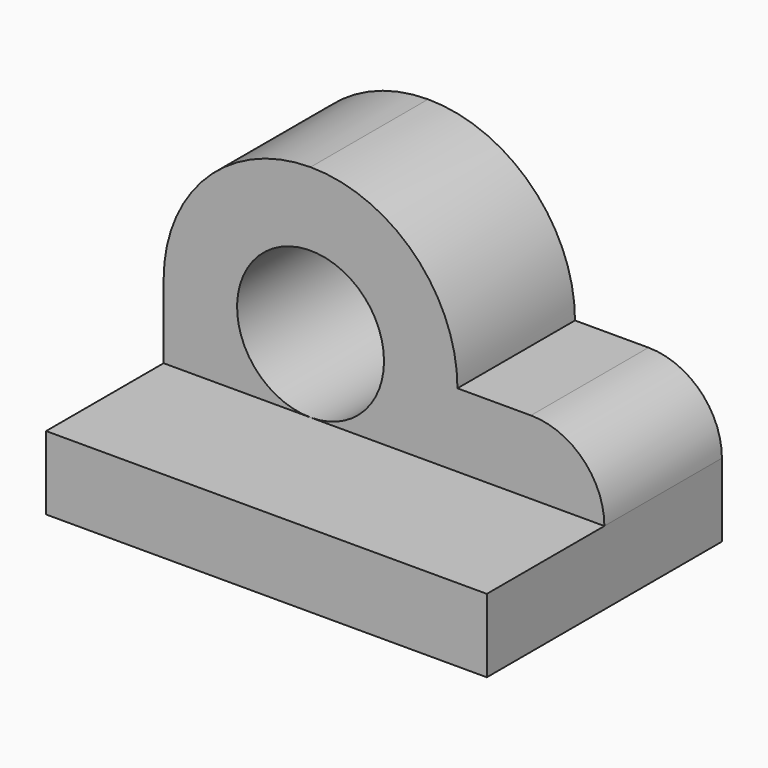
from build123d import *

# Parameters (mm, degrees)
F0_W     = 60
F0_H     = 10
F1_DEPTH = 40
F2_W     = 60
F2_H     = 20
F3_DEPTH = 10
F4_W     = 40
F4_H     = 20
F5_DEPTH = 20
F6_R     = 19.99999
F7_R     = 10
F8_R     = 10
F9_DEPTH = 25


# Not quite as in the source:
# - a fillet or chamfer is up to 0.001 mm smaller than in the source, because OpenCascade refuses the exact size


with BuildPart() as f1:
    # F0 (on Front) → F1 (new body)
    with BuildSketch(Plane.XZ):
        with Locations((30, 5)):
            Rectangle(F0_W, F0_H)
    extrude(amount=F1_DEPTH)

    # F2 (on face) → F3 (join)
    with BuildSketch(Plane.XY.offset(10)):
        with Locations((30, -10)):
            Rectangle(F2_W, F2_H)
    extrude(amount=F3_DEPTH)

    # F4 (on face) → F5 (join)
    with BuildSketch(Plane.XY.offset(20)):
        with Locations((20, -10)):
            Rectangle(F4_W, F4_H)
    extrude(amount=F5_DEPTH)

    # F6 (radius 20 in the source; OpenCascade refuses exactly that, so slightly less here)
    f6_edges = [f1.edges().sort_by_distance(p)[0] for p in [
        (0, -10, 40),
        (40, -10, 40),
    ]]
    fillet(f6_edges, radius=F6_R)

    # F7
    f7_edges = [f1.edges().sort_by_distance(p)[0] for p in [
        (60, -10, 20),
    ]]
    fillet(f7_edges, radius=F7_R)

    # F8 (on face) → F9 (cut)
    with BuildSketch(Plane.XZ.offset(20)):
        with Locations((20, 20)):
            Circle(F8_R)
    extrude(amount=-F9_DEPTH, mode=Mode.SUBTRACT)


solid = f1.part
